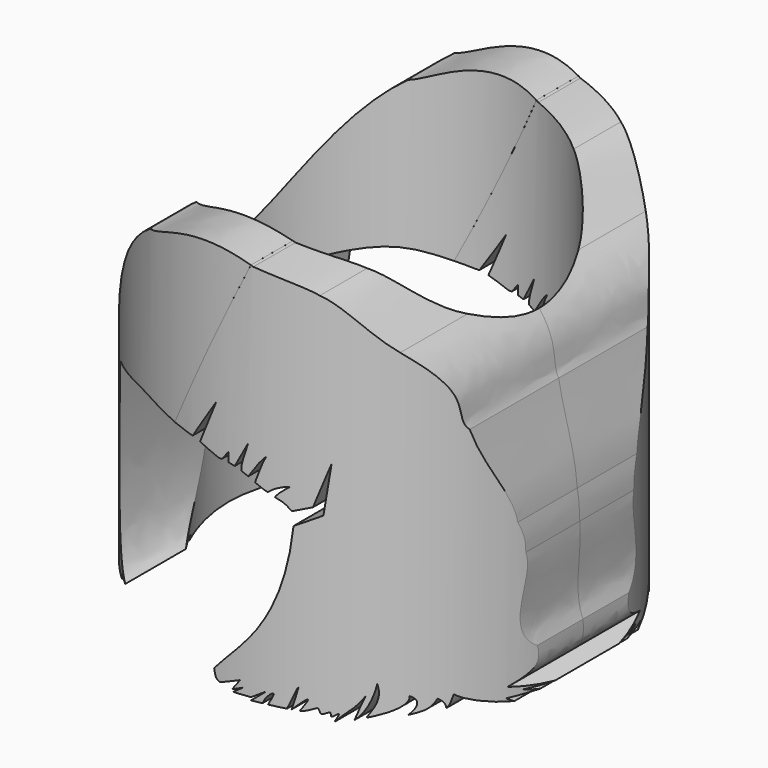
from build123d import *

# Parameters (mm, degrees)
F0_R     = 12
F0_R_2   = 9
F1_DEPTH = 27.6
F2_W     = 28.2279141247
F2_H     = 30.2608710481
F3_DEPTH = 16.4
F5_DEPTH = 19.6


with BuildPart() as f1:
    # F0 (on Top) → F1 (new body)
    with BuildSketch(Plane.XY):
        Circle(F0_R)
        Circle(F0_R_2, mode=Mode.SUBTRACT)
    extrude(amount=-F1_DEPTH)

    # F2 (on Front) → F3 (cut, symmetric)
    with BuildSketch(Plane.XZ):
        with Locations((-0.3088144585, -13.4869223111)):
            Rectangle(F2_W, F2_H)
        with BuildLine():
            add(Edge.make_bspline(
                [(-4.7268979251, -2.6836635079), (-3.774828976, -2.6345571969), (-1.3583082473, -0.6711342139), (1.9063265063, -2.1388111636)],
                knots=[0, 0, 0, 0, 6.6555638705, 6.6555638705, 6.6555638705, 6.6555638705], degree=3))
            add(Edge.make_bspline(
                [(1.9063265063, -2.1388111636), (3.1286855228, -2.3624252062), (4.4190459885, -2.6457584463), (5.0067203119, -2.9805628583)],
                knots=[0, 0, 0, 0, 3.2126294006, 3.2126294006, 3.2126294006, 3.2126294006], degree=3))
            add(Edge.make_bspline(
                [(8.0554401502, -5.7192435488), (7.0392002041, -4.8063499853), (6.0401847586, -3.3939480782), (5.0067203119, -2.9805628583)],
                knots=[0, 0, 0, 0, 4.0981782022, 4.0981782022, 4.0981782022, 4.0981782022], degree=3))
            add(Edge.make_bspline(
                [(10.1223699749, -9.9564483389), (9.6056377515, -9.1296769679), (10.4324091226, -7.9411929473), (8.0554401502, -5.7192435488)],
                knots=[0, 0, 0, 0, 4.7144568439, 4.7144568439, 4.7144568439, 4.7144568439], degree=3))
            add(Edge.make_bspline(
                [(11.2006255345, -15.2145396242), (11.0921614432, -13.3933477802), (10.4618292538, -11.8898905502), (10.1223699749, -9.9564483389)],
                knots=[0.9009982526, 0.9009982526, 0.9009982526, 0.9009982526, 6.295021157, 6.295021157, 6.295021157, 6.295021157], degree=3))
            add(Edge.make_bspline(
                [(11.2006255345, -15.2145396242), (11.2758269534, -15.6726706773), (11.3471858203, -16.0354096442), (11.3457852497, -16.8596208984)],
                knots=[0, 0, 0, 0, 1.6514732035, 1.6514732035, 1.6514732035, 1.6514732035], degree=3))
            add(Edge.make_bspline(
                [(11.5339493159, -21.7919425752), (10.9077528305, -20.4053621673), (11.5082064192, -18.4362875254), (11.3457852497, -16.8596208984)],
                knots=[0, 0, 0, 0, 4.8855830955, 4.8855830955, 4.8855830955, 4.8855830955], degree=3))
            add(Edge.make_bspline(
                [(10.9939305112, -23.4824754298), (11.4318979904, -23.1129396707), (11.6235082969, -22.9213293642), (11.5339493159, -21.7919425752)],
                knots=[0, 0, 0, 0, 1.7746891677, 1.7746891677, 1.7746891677, 1.7746891677], degree=3))
            Line((10.9939305112, -23.4824754298), (11.7740593851, -23.9067561924))
            Line((11.7740593851, -23.9067561924), (11.2713351846, -23.8113421947))
            Line((11.2713351846, -23.8113421947), (11.5794669837, -24.046972394))
            Line((11.5794669837, -24.046972394), (10.9668290243, -24.046972394))
            Line((10.9668290243, -24.046972394), (11.1335823312, -24.2898538709))
            add(Edge.make_bspline(
                [(9.7016766667, -23.3582090586), (9.9771823734, -23.702589795), (10.6768226251, -24.0832231939), (11.1335823312, -24.2898538709)],
                knots=[0, 0, 0, 0, 1.708307902, 1.708307902, 1.708307902, 1.708307902], degree=3))
            add(Edge.make_bspline(
                [(9.4877975062, -24.0179728717), (9.6291759983, -23.8367188722), (9.6328000848, -23.5600049297), (9.7016766667, -23.3582090586)],
                knots=[0, 0, 0, 0, 0.6935651262, 0.6935651262, 0.6935651262, 0.6935651262], degree=3))
            add(Edge.make_bspline(
                [(9.2340419069, -23.4814602882), (9.4297956675, -23.6409641802), (9.4877975062, -23.8838437945), (9.4877975062, -24.0179728717)],
                knots=[0, 0, 0, 0, 0.5934961301, 0.5934961301, 0.5934961301, 0.5934961301], degree=3))
            add(Edge.make_bspline(
                [(8.3241472021, -24.213725701), (8.7954076007, -24.0687225014), (9.0455375612, -24.0034721792), (9.2340419069, -23.4814602882)],
                knots=[0, 0, 0, 0, 1.1679559104, 1.1679559104, 1.1679559104, 1.1679559104], degree=3))
            add(Edge.make_bspline(
                [(8.3676483482, -23.2530813664), (8.7990323082, -23.5285870731), (8.5742780939, -23.9345952868), (8.3241472021, -24.213725701)],
                knots=[0, 0, 0, 0, 0.9616287679, 0.9616287679, 0.9616287679, 0.9616287679], degree=3))
            add(Edge.make_bspline(
                [(6.8582138047, -24.3477188051), (7.004532963, -24.2867525667), (8.4250476211, -23.9422935992), (8.3676483482, -23.2530813664)],
                knots=[0, 0, 0, 0, 1.8645706646, 1.8645706646, 1.8645706646, 1.8645706646], degree=3))
            add(Edge.make_bspline(
                [(7.2555966932, -22.6150569635), (7.46288209, -23.3984743374), (7.1020787582, -23.9118095487), (6.8582138047, -24.3477188051)],
                knots=[0, 0, 0, 0, 1.7776473827, 1.7776473827, 1.7776473827, 1.7776473827], degree=3))
            add(Edge.make_bspline(
                [(6.4121595756, -24.4840684984), (6.8978415802, -24.0825153887), (7.1843834594, -23.1192484498), (7.2555966932, -22.6150569635)],
                knots=[0, 0, 0, 0, 2.0505097632, 2.0505097632, 2.0505097632, 2.0505097632], degree=3))
            add(Edge.make_bspline(
                [(6.8307660939, -23.2388981105), (6.6571710831, -23.6520501068), (6.5590729908, -24.0694243167), (6.4121595756, -24.4840684984)],
                knots=[0.2349726848, 0.2349726848, 0.2349726848, 0.2349726848, 1.5546772505, 1.5546772505, 1.5546772505, 1.5546772505], degree=3))
            add(Edge.make_bspline(
                [(5.6114532053, -24.6555991471), (6.0094881337, -24.1619623488), (6.4956751909, -23.892864126), (6.8307660939, -23.2388981105)],
                knots=[0, 0, 0, 0, 1.9023621726, 1.9023621726, 1.9023621726, 1.9023621726], degree=3))
            add(Edge.make_bspline(
                [(5.6114532053, -24.6555991471), (5.7246088606, -24.4345325268), (5.9344108602, -24.0249936614), (5.4108265301, -24.5638843492), (5.5264887917, -24.0342632444), (4.9763764137, -24.5038601943), (4.9986215308, -24.0857861936), (4.9042264, -24.0385886282)],
                knots=[0, 0, 0, 0, 0.2349074199, 0.4341103406, 0.5897608658, 0.8032421322, 1, 1, 1, 1], degree=3))
            add(Edge.make_bspline(
                [(4.9042264, -24.0385886282), (4.6477856425, -24.1266911228), (4.4369692914, -24.2934562266), (4.1349041276, -24.3028961122)],
                knots=[0, 0, 0, 0, 0.8134587912, 0.8134587912, 0.8134587912, 0.8134587912], degree=3))
            add(Edge.make_bspline(
                [(4.1349041276, -24.3028961122), (4.3319962706, -23.9949038662), (4.7559626748, -23.332379409), (4.1066446434, -23.964587104), (3.7591794971, -24.3028961122)],
                knots=[0, 0, 0, 0, 0.4648767946, 1, 1, 1, 1], degree=3))
            add(Edge.make_bspline(
                [(3.7591794971, -24.3028961122), (3.9282517112, -23.7143626433), (4.2710469307, -22.521106491), (3.7923810069, -23.7036184235), (3.5498009529, -24.3028961122)],
                knots=[0, 0, 0, 0, 0.4932163709, 1, 1, 1, 1], degree=3))
            add(Edge.make_bspline(
                [(3.5498009529, -24.3028961122), (3.2479996638, -24.2975149304), (2.9461983747, -24.2921337485), (2.6443970855, -24.2867525667)],
                knots=[0, 0, 0, 0, 0.9055477774, 0.9055477774, 0.9055477774, 0.9055477774], degree=3))
            add(Edge.make_bspline(
                [(2.6443970855, -24.2867525667), (2.7937771075, -23.9847798557), (3.1601787014, -23.3746710663), (2.5089443661, -23.9090491086), (2.3703414481, -24.2867525667)],
                knots=[0, 0, 0, 0, 0.4754339891, 1, 1, 1, 1], degree=3))
            Line((2.3703414481, -24.2867525667), (1.7888071015, -24.2867525667))
            Line((1.7888071015, -24.2867525667), (2.5538711343, -23.6419886351))
            Line((2.5538711343, -23.6419886351), (1.7888071015, -24.1220295429))
            Line((1.7888071015, -24.1220295429), (0.8437280194, -24.1220295429))
            Line((0.8437280194, -24.1220295429), (1.3437698362, -23.761998862))
            Line((1.3437698362, -23.761998862), (0.7741009467, -24.0030623972))
            Line((0.7741009467, -24.0030623972), (1.2151370756, -23.4096515924))
            Line((1.2151370756, -23.4096515924), (0.0912897687, -23.8611114358))
            add(Edge.make_bspline(
                [(-0.2446891212, -23.2431141408), (-0.1684888557, -23.69055897), (-0.136988092, -23.7598605454), (0.0912897687, -23.8611114358)],
                knots=[0, 0, 0, 0, 0.7034219722, 0.7034219722, 0.7034219722, 0.7034219722], degree=3))
            add(Edge.make_bspline(
                [(-0.2446891212, -23.2431141408), (1.2196582172, -21.5136555109), (3.3710643509, -20.2898978744), (3.8490038716, -14.9241725775)],
                knots=[0.2648466476, 0.2648466476, 0.2648466476, 0.2648466476, 9.4620957656, 9.4620957656, 9.4620957656, 9.4620957656], degree=3))
            Line((3.8490038716, -14.9241725775), (5.157333333, -14.1847999766))
            Line((5.157333333, -14.1847999766), (5.4971566424, -11.5039721131))
            Line((5.4971566424, -11.5039721131), (4.7134207562, -13.8206714764))
            Line((4.7134207562, -13.8206714764), (3.7684009876, -14.1847999766))
            add(Edge.make_bspline(
                [(3.7684009876, -14.1847999766), (3.5621593706, -13.972424902), (3.4722534474, -13.822581619), (2.9777705204, -13.6352777481)],
                knots=[0, 0, 0, 0, 0.9628453746, 0.9628453746, 0.9628453746, 0.9628453746], degree=3))
            add(Edge.make_bspline(
                [(2.9777705204, -13.6352777481), (3.0751687009, -13.4704494849), (3.2924413681, -13.2531775162), (3.6970181391, -12.960982509)],
                knots=[0, 0, 0, 0, 0.9858961439, 0.9858961439, 0.9858961439, 0.9858961439], degree=3))
            add(Edge.make_bspline(
                [(3.6970181391, -12.960982509), (3.3523787279, -13.0134280771), (2.9253254179, -13.1857478991), (2.6256390847, -13.4629579261)],
                knots=[0, 0, 0, 0, 1.1831451295, 1.1831451295, 1.1831451295, 1.1831451295], degree=3))
            add(Edge.make_bspline(
                [(2.6256390847, -13.4629579261), (2.3945157489, -13.3555057132), (2.1919206062, -13.233240902), (1.9934395976, -13.111157654)],
                knots=[0, 0, 0, 0, 0.7643507945, 0.7643507945, 0.7643507945, 0.7643507945], degree=3))
            add(Edge.make_bspline(
                [(1.9934395976, -13.111157654), (1.8763583848, -13.0391424278), (1.7607087498, -12.9671903794), (1.6414794579, -12.8983792136)],
                knots=[0.7643507945, 0.7643507945, 0.7643507945, 0.7643507945, 1.2152307988, 1.2152307988, 1.2152307988, 1.2152307988], degree=3))
            add(Edge.make_bspline(
                [(1.6414794579, -12.8983792136), (1.5260543955, -12.8317635944), (1.407274463, -12.7680916241), (1.2805929613, -12.7101557077)],
                knots=[1.2152307988, 1.2152307988, 1.2152307988, 1.2152307988, 1.6517246483, 1.6517246483, 1.6517246483, 1.6517246483], degree=3))
            add(Edge.make_bspline(
                [(1.2805929613, -12.7101557077), (1.1690745515, -12.6591544078), (1.0514329187, -12.6125981916), (0.9245663878, -12.5723919871)],
                knots=[1.6517246483, 1.6517246483, 1.6517246483, 1.6517246483, 2.0359725402, 2.0359725402, 2.0359725402, 2.0359725402], degree=3))
            add(Edge.make_bspline(
                [(0.9245663878, -12.5723919871), (0.8184306264, -12.538755723), (0.7058384577, -12.5095637641), (0.5849737791, -12.4859314895)],
                knots=[2.0359725402, 2.0359725402, 2.0359725402, 2.0359725402, 2.3574319688, 2.3574319688, 2.3574319688, 2.3574319688], degree=3))
            add(Edge.make_bspline(
                [(0.5849737791, -12.4859314895), (0.4647580639, -12.4624261045), (0.3363584363, -12.4444208604), (0.1979878909, -12.4330132662)],
                knots=[2.3574319688, 2.3574319688, 2.3574319688, 2.3574319688, 2.6771653726, 2.6771653726, 2.6771653726, 2.6771653726], degree=3))
            add(Edge.make_bspline(
                [(0.1979878909, -12.4330132662), (0.1341712413, -12.4277520711), (0.068233713, -12.4238942387), (0, -12.4215474352)],
                knots=[2.6771653726, 2.6771653726, 2.6771653726, 2.6771653726, 2.8246267742, 2.8246267742, 2.8246267742, 2.8246267742], degree=3))
            add(Edge.make_bspline(
                [(0, -12.4215474352), (-0.3476848482, -12.304156532), (-0.7252554593, -12.1192681927), (-1.0969288382, -11.9882814159)],
                knots=[0, 0, 0, 0, 1.1516303564, 1.1516303564, 1.1516303564, 1.1516303564], degree=3))
            add(Edge.make_bspline(
                [(-1.0969288382, -11.9882814159), (-1.2564957607, -11.932046135), (-1.4149757295, -11.8857457697), (-1.5695372161, -11.8589866906)],
                knots=[1.1516303564, 1.1516303564, 1.1516303564, 1.1516303564, 1.6460486341, 1.6460486341, 1.6460486341, 1.6460486341], degree=3))
            add(Edge.make_bspline(
                [(-1.5695372161, -11.8589866906), (-1.6422061979, -11.8464055809), (-1.7140089891, -11.8381441228), (-1.7846513074, -11.8352007121)],
                knots=[1.6460486341, 1.6460486341, 1.6460486341, 1.6460486341, 1.8785054615, 1.8785054615, 1.8785054615, 1.8785054615], degree=3))
            add(Edge.make_bspline(
                [(-8.5255475715, -11.684906669), (-4.8105460592, -10.8509846032), (-5.0558447838, -11.3003198057), (-1.7846513074, -11.8352007121)],
                knots=[0, 0, 0, 0, 6.742571523, 6.742571523, 6.742571523, 6.742571523], degree=3))
            add(Edge.make_bspline(
                [(-8.5255475715, -11.684906669), (-8.7895141914, -14.4368428737), (-9.4252461568, -21.2603565305), (-7.4998005293, -22.3847813904)],
                knots=[0, 0, 0, 0, 10.7489290652, 10.7489290652, 10.7489290652, 10.7489290652], degree=3))
            add(Edge.make_bspline(
                [(-7.4998005293, -22.3847813904), (-7.7263408651, -22.3847813904), (-8.0485977232, -22.1790745854), (-8.1794215366, -22.3847813904)],
                knots=[0, 0, 0, 0, 0.6796210073, 0.6796210073, 0.6796210073, 0.6796210073], degree=3))
            add(Edge.make_bspline(
                [(-8.1794215366, -22.3847813904), (-8.1614833325, -22.4459320307), (-8.1124790013, -22.4710963666), (-8.060333319, -22.5109755993)],
                knots=[0, 0, 0, 0, 0.1735136361, 0.1735136361, 0.1735136361, 0.1735136361], degree=3))
            add(Edge.make_bspline(
                [(-8.060333319, -22.5109755993), (-8.6952047423, -22.5810911506), (-9.3064047396, -22.5175898522), (-10.0207952783, -22.0651421696)],
                knots=[0, 0, 0, 0, 2.0105169834, 2.0105169834, 2.0105169834, 2.0105169834], degree=3))
            add(Edge.make_bspline(
                [(-10.0207952783, -22.0651421696), (-9.9365506321, -22.3516467959), (-9.8865460604, -22.5416626781), (-9.9115483463, -22.5916672498)],
                knots=[0, 0, 0, 0, 0.5377392976, 0.5377392976, 0.5377392976, 0.5377392976], degree=3))
            add(Edge.make_bspline(
                [(-10.5966059491, -22.1016258001), (-10.3682534148, -22.26497295), (-10.1965721697, -22.3416462541), (-9.9115483463, -22.5916672498)],
                knots=[0, 0, 0, 0, 0.8422853089, 0.8422853089, 0.8422853089, 0.8422853089], degree=3))
            add(Edge.make_bspline(
                [(-10.5966059491, -22.1016258001), (-10.6327697677, -22.1375252092), (-10.6477964683, -22.1751129903), (-10.6537198208, -22.2096662847)],
                knots=[0, 0, 0, 0, 0.1026326122, 0.1026326122, 0.1026326122, 0.1026326122], degree=3))
            add(Edge.make_bspline(
                [(-10.6537198208, -22.2096662847), (-10.7321301777, -22.2111559441), (-10.8105954903, -22.2126361825), (-10.8890058473, -22.2141258419)],
                knots=[0, 0, 0, 0, 0.2353282854, 0.2353282854, 0.2353282854, 0.2353282854], degree=3))
            add(Edge.make_bspline(
                [(-10.8890058473, -22.2141258419), (-11.2732192501, -21.7026863247), (-11.5914214402, -21.6226577759), (-11.7577118799, -20.6679441035)],
                knots=[0, 0, 0, 0, 1.7735072989, 1.7735072989, 1.7735072989, 1.7735072989], degree=3))
            add(Edge.make_bspline(
                [(-11.7577118799, -20.6679441035), (-10.5845741928, -15.8115122467), (-9.6302367747, -5.9970174916), (-4.7268979251, -2.6836635079)],
                knots=[0, 0, 0, 0, 19.3097564305, 19.3097564305, 19.3097564305, 19.3097564305], degree=3))
        make_face(mode=Mode.SUBTRACT)
        with BuildLine():
            Line((-0.1196217127, -9.6230907366), (-1.5695372161, -11.8589866906))
            add(Edge.make_bspline(
                [(-1.0969288382, -11.9882814159), (-1.2564957607, -11.932046135), (-1.4149757295, -11.8857457697), (-1.5695372161, -11.8589866906)],
                knots=[1.1516303564, 1.1516303564, 1.1516303564, 1.1516303564, 1.6460486341, 1.6460486341, 1.6460486341, 1.6460486341], degree=3))
            Line((-1.0969288382, -11.9882814159), (-0.1196217127, -9.6230907366))
        make_face()
        with BuildLine():
            add(Edge.make_bspline(
                [(2.5582097005, -11.6573469713), (2.116171876, -12.0844002813), (1.9486934799, -12.4818648896), (1.6414794579, -12.8983792136)],
                knots=[0, 0, 0, 0, 1.5429048461, 1.5429048461, 1.5429048461, 1.5429048461], degree=3))
            add(Edge.make_bspline(
                [(1.9934395976, -13.111157654), (1.8763583848, -13.0391424278), (1.7607087498, -12.9671903794), (1.6414794579, -12.8983792136)],
                knots=[0.7643507945, 0.7643507945, 0.7643507945, 0.7643507945, 1.2152307988, 1.2152307988, 1.2152307988, 1.2152307988], degree=3))
            add(Edge.make_bspline(
                [(2.5582097005, -11.6573469713), (2.288491698, -12.1443374082), (2.1815162113, -12.6268468761), (1.9934395976, -13.111157654)],
                knots=[0, 0, 0, 0, 1.5596572605, 1.5596572605, 1.5596572605, 1.5596572605], degree=3))
        make_face()
        with BuildLine():
            Line((1.6298081789, -11.2283160485), (0.9245663878, -12.5723919871))
            add(Edge.make_bspline(
                [(1.2805929613, -12.7101557077), (1.1690745515, -12.6591544078), (1.0514329187, -12.6125981916), (0.9245663878, -12.5723919871)],
                knots=[1.6517246483, 1.6517246483, 1.6517246483, 1.6517246483, 2.0359725402, 2.0359725402, 2.0359725402, 2.0359725402], degree=3))
            add(Edge.make_bspline(
                [(1.6298081789, -11.2283160485), (1.5134031063, -11.7222626016), (1.2401558924, -12.3029723763), (1.2805929613, -12.7101557077)],
                knots=[0, 0, 0, 0, 1.5224322788, 1.5224322788, 1.5224322788, 1.5224322788], degree=3))
        make_face()
        with BuildLine():
            Line((0.5849737791, -11.9458024747), (0.1979878909, -12.4330132662))
            add(Edge.make_bspline(
                [(0.5849737791, -12.4859314895), (0.4647580639, -12.4624261045), (0.3363584363, -12.4444208604), (0.1979878909, -12.4330132662)],
                knots=[2.3574319688, 2.3574319688, 2.3574319688, 2.3574319688, 2.6771653726, 2.6771653726, 2.6771653726, 2.6771653726], degree=3))
            Line((0.5849737791, -12.4859314895), (0.5849737791, -11.9458024747))
        make_face()
    extrude(amount=F3_DEPTH, both=True, mode=Mode.SUBTRACT)

    # F4 (on Front) → F5 (cut, symmetric)
    with BuildSketch(Plane.XZ):
        Polygon((-3.9394633154, -14.0837163814), (2.682594342, -0.1882515885), (2.681594342, -0.1882515885), (-3.9404633154, -14.0837163814), align=None)
    extrude(amount=F5_DEPTH, both=True, mode=Mode.SUBTRACT)


solid = f1.part
